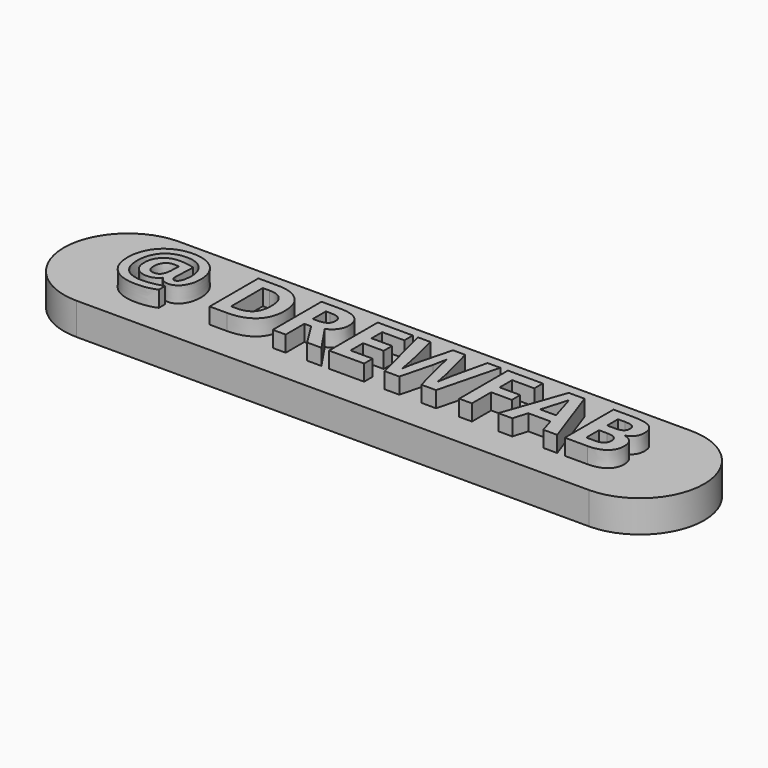
from build123d import *

# Parameters (mm, degrees)
F1_DEPTH     = 3.175
F2_TEXT_SIZE = 8.4565364407
F3_DEPTH     = 1.5875


# Not quite as in the source:
# - Text() gives the source's letters only with a copy of the font that has no kerning and outlines rounded to 1/6400 em; it was checked with that copy


with BuildPart() as f1:
    # F0 (on Top) → F1 (new body)
    with BuildSketch(Plane.XY):
        with BuildLine():
            ThreePointArc((25.4, -6.35), (31.75, 0), (25.4, 6.35))
            Line((25.4, 6.35), (-25.4, 6.35))
            ThreePointArc((-25.4, 6.35), (-31.75, 0), (-25.4, -6.35))
            Line((-25.4, -6.35), (25.4, -6.35))
        make_face()
    extrude(amount=F1_DEPTH)

    # F2 (on face) → F3 (join)
    with BuildSketch(Plane.XY.offset(3.175)):
        with Locations((-25.4, -3.0443531187)):
            Text('@ DREWFAB', F2_TEXT_SIZE, font='Open Sans', font_style=FontStyle.BOLD, text_align=(TextAlign.LEFT, TextAlign.BOTTOM))
    extrude(amount=F3_DEPTH)


solid = f1.part
